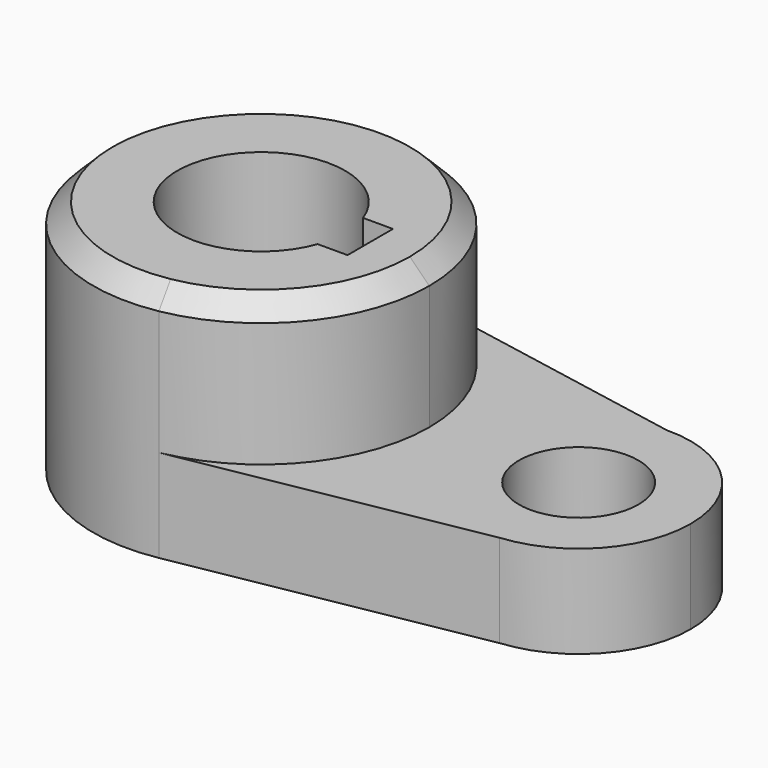
from build123d import *

# Parameters (mm, degrees)
F0_R     = 10.16
F1_DEPTH = 15.7734
F2_DEPTH = 40.2336
F3_SIZE  = 3.302


# Not quite as in the source:
# - a feature names something its author has since deleted; it is built from what else it names


with BuildPart() as f1:
    # F0 (on Top) → F1 (new body)
    with BuildSketch(Plane.XY):
        with BuildLine():
            ThreePointArc((5.2429423077, 28.0898946413), (21.9812158608, 18.258060529), (28.575, 0))
            ThreePointArc((28.575, 0), (21.9291125509, -18.3206071879), (5.0828111824, -28.1193110777))
            Line((5.0828111824, -28.1193110777), (55.6786843639, -18.9736648961))
            ThreePointArc((55.6786843639, -18.9736648961), (34.9510761924, -0.9964050199), (53.687254757, 19.0478267179))
            Line((53.687254757, 19.0478267179), (5.2429423077, 28.0898946413))
        make_face()
        with BuildLine():
            ThreePointArc((73.025, 0), (67.3432637826, 13.5717361984), (53.687254757, 19.0478267179))
            ThreePointArc((53.687254757, 19.0478267179), (34.9510761924, -0.9964050199), (55.6786843639, -18.9736648961))
            ThreePointArc((55.6786843639, -18.9736648961), (68.0348308513, -12.8539354454), (73.025, 0))
        make_face()
        with Locations((53.975, 0)):
            Circle(F0_R, mode=Mode.SUBTRACT)
    extrude(amount=F1_DEPTH)

    # F0 (on Top) → F2 (join)
    with BuildSketch(Plane.XY):
        with BuildLine():
            ThreePointArc((5.0828111824, -28.1193110777), (21.9291125509, -18.3206071879), (28.575, 0))
            ThreePointArc((28.575, 0), (21.9812158608, 18.258060529), (5.2429423077, 28.0898946413))
            ThreePointArc((5.2429423077, 28.0898946413), (-28.5748840448, 0.0814053193), (5.0828111824, -28.1193110777))
        make_face()
        with BuildLine():
            ThreePointArc((13.4477648793, -4.826), (-14.2875, 0), (13.4477648793, 4.826))
            Line((13.4477648793, 4.826), (18.5293, 4.826))
            Line((18.5293, 4.826), (18.5293, 0))
            Line((18.5293, 0), (18.5293, -4.826))
            Line((18.5293, -4.826), (13.4477648793, -4.826))
        make_face(mode=Mode.SUBTRACT)
    extrude(amount=F2_DEPTH)

    # F3
    f3_edges = [f1.edges().sort_by_distance(p)[0] for p in [
        (-5.082811, 28.119311, 40.2336),
    ]]
    chamfer(f3_edges, length=F3_SIZE)


solid = f1.part
